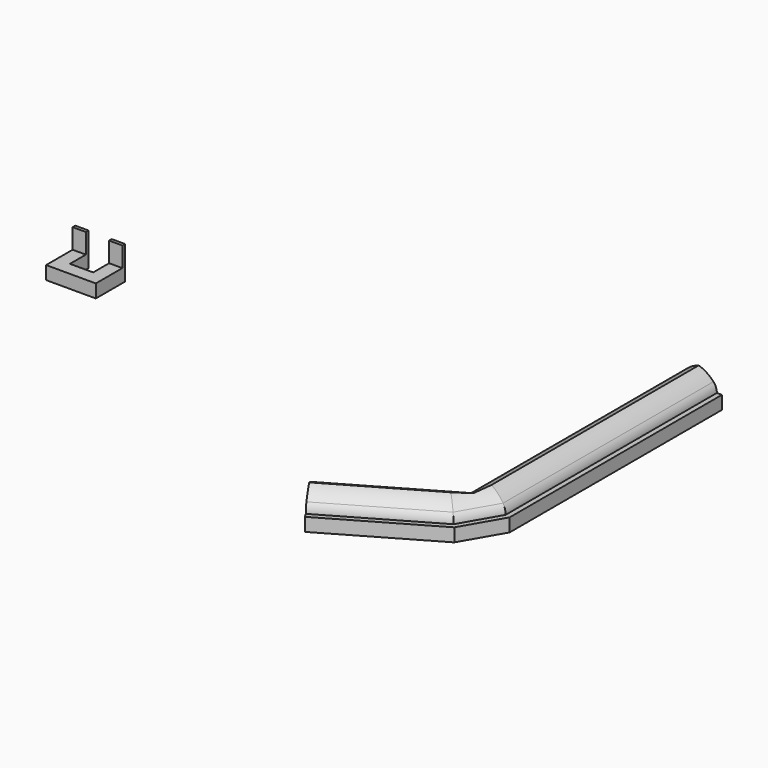
from build123d import *

# Parameters (mm, degrees)
F0_W         = 7
F0_H         = 40
F1_DEPTH     = 5
F2_T1_DEPTH  = 32
F2_T3_DEPTH  = 42.8011414996
F2_T5_DEPTH  = 65
F2_T10_DEPTH = 65
F2_T15_DEPTH = 42.8011414996
F2_T21_DEPTH = 65
F2_T25_DEPTH = 42.8011414996
F3_R         = 2
F4_DEPTH     = 2
F0_W_2       = 2
F0_H_2       = 0.5
F5_DEPTH     = 5


# Not quite as in the source:
# - a fillet or chamfer that OpenCascade refuses, or shapes differently, is made with other operations: its cross-section is extruded or revolved along the edge and cut away or added


with BuildPart() as f1:
    # F0 (on Top) → F1 (new body)
    with BuildSketch(Plane.XY):
        Polygon((30.4447099417, -16.7805150867), (26.9447099417, -10.7183372602), (11.5284691868, -19.61890801), (15.0284691868, -25.6810858365), align=None)
        Polygon((33.9447099417, -10.7183372602), (26.9447099417, -10.7183372602), (30.4447099417, -16.7805150867), align=None)
        with Locations((30.4447099417, 9.2816627398)):
            Rectangle(F0_W, F0_H)
    extrude(amount=F1_DEPTH)

    # F2: fillet of radius 5 on 5 edges, made by hand

    # F2_s2 → F2_t1 (cut)
    with BuildSketch(Plane(origin=(-5.9049986914, -10.2277577521, 0), x_dir=(0, 0, 1), z_dir=(0.5, 0.8660254038, 0))):
        with BuildLine():
            ThreePointArc((0, 34.7561497637), (3.5355339059, 33.2916836697), (5, 29.7561497637))
            Line((5, 29.7561497637), (5, 34.7561497637))
            Line((5, 34.7561497637), (0, 34.7561497637))
        make_face()
    extrude(amount=F2_T1_DEPTH, mode=Mode.SUBTRACT)

    # F2_s4 → F2_t3 (cut)
    with BuildSketch(Plane(origin=(-10.6742020228, -6.1627534112, 0), x_dir=(0, 0, 1), z_dir=(0.8660254038, 0.5, 0))):
        with BuildLine():
            ThreePointArc((0, 29.7547073245), (3.5355339059, 28.2902412305), (5, 24.7547073245))
            Line((5, 24.7547073245), (5, 29.7547073245))
            Line((5, 29.7547073245), (0, 29.7547073245))
        make_face()
    extrude(amount=F2_T3_DEPTH, mode=Mode.SUBTRACT)

    # F2_s6 → F2_t5 (cut)
    with BuildSketch(Plane.XZ.offset(-41.7816627398)):
        with BuildLine():
            ThreePointArc((33.9447099417, 0), (32.4802438477, 3.5355339059), (28.9447099417, 5))
            Line((28.9447099417, 5), (33.9447099417, 5))
            Line((33.9447099417, 5), (33.9447099417, 0))
        make_face()
    extrude(amount=F2_T5_DEPTH, mode=Mode.SUBTRACT)


with BuildPart() as f2_tool8:
    # F2_s9 → F2_t10 (new body)
    with BuildSketch(Plane.XZ.offset(-41.7816627398)):
        with BuildLine():
            ThreePointArc((26.9447099417, 0), (28.4091760358, 3.5355339059), (31.9447099417, 5))
            Line((31.9447099417, 5), (26.9447099417, 5))
            Line((26.9447099417, 5), (26.9447099417, 0))
        make_face()
    extrude(amount=F2_T10_DEPTH)

    split(bisect_by=Plane(origin=(11.3773536623, -19.7061545987, 0), x_dir=(0, 0, 1), z_dir=(-0.5, 0.8660254038, 0)), keep=Keep.TOP)


with BuildPart() as f1_1:
    add(f1.part)

    # F2_t7: cut F2_tool8
    add(f2_tool8.part, mode=Mode.SUBTRACT)


with BuildPart() as f2_tool13:
    # F2_s14 → F2_t15 (new body)
    with BuildSketch(Plane(origin=(26.3926738268, 15.2378173385, 0), x_dir=(0, 0, 1), z_dir=(-0.8660254038, -0.5, 0))):
        with BuildLine():
            ThreePointArc((0, -22.7547073245), (3.5355339059, -24.2191734186), (5, -27.7547073245))
            Line((5, -27.7547073245), (5, -22.7547073245))
            Line((5, -22.7547073245), (0, -22.7547073245))
        make_face()
    extrude(amount=F2_T15_DEPTH)

    split(bisect_by=Plane.YZ.offset(26.9447099417), keep=Keep.BOTTOM)


with BuildPart() as f1_2:
    add(f1_1.part)

    # F2_t12: cut F2_tool13
    add(f2_tool13.part, mode=Mode.SUBTRACT)


with BuildPart() as f2_tool19:
    # F2_s20 → F2_t21 (new body)
    with BuildSketch(Plane.XZ.offset(-41.7816627398)):
        with BuildLine():
            ThreePointArc((26.9447099417, 0), (28.4091760358, 3.5355339059), (31.9447099417, 5))
            Line((31.9447099417, 5), (26.9447099417, 5))
            Line((26.9447099417, 5), (26.9447099417, 0))
        make_face()
    extrude(amount=F2_T21_DEPTH)

    split(bisect_by=Plane(origin=(11.3773536623, -19.7061545987, 0), x_dir=(0, 0, 1), z_dir=(0.5, -0.8660254038, 0)), keep=Keep.TOP)


with BuildPart() as f2_tool23:
    # F2_s24 → F2_t25 (new body)
    with BuildSketch(Plane(origin=(26.3926738268, 15.2378173385, 0), x_dir=(0, 0, 1), z_dir=(-0.8660254038, -0.5, 0))):
        with BuildLine():
            ThreePointArc((0, -22.7547073245), (3.5355339059, -24.2191734186), (5, -27.7547073245))
            Line((5, -27.7547073245), (5, -22.7547073245))
            Line((5, -22.7547073245), (0, -22.7547073245))
        make_face()
    extrude(amount=F2_T25_DEPTH)

    split(bisect_by=Plane.YZ.offset(26.9447099417), keep=Keep.TOP)


with BuildPart() as f2_tool19_1:
    add(f2_tool19.part)

    # F2_t27: intersect F2_tool23
    add(f2_tool23.part, mode=Mode.INTERSECT)


with BuildPart() as f1_3:
    add(f1_2.part)

    # F2_t17: cut F2_tool19
    add(f2_tool19_1.part, mode=Mode.SUBTRACT)

    # F3
    f3_edges = [f1_3.edges().sort_by_distance(p)[0] for p in [
        (13.278469, -22.649997, 0),
        (22.73659, -21.2308, 0),
        (19.23659, -15.168623, 0),
        (26.94471, 9.281663, 0),
        (33.94471, 9.281663, 0),
        (32.19471, -13.749426, 0),
        (30.44471, 29.281663, 0),
    ]]
    fillet(f3_edges, radius=F3_R)

    # F0 (on Top) → F4 (join)
    with BuildSketch(Plane.XY):
        with Locations((30.4447099417, 9.2816627398)):
            Rectangle(F0_W, F0_H)
        Polygon((30.4447099417, -16.7805150867), (26.9447099417, -10.7183372602), (11.5284691868, -19.61890801), (15.0284691868, -25.6810858365), align=None)
        Polygon((33.9447099417, -10.7183372602), (26.9447099417, -10.7183372602), (30.4447099417, -16.7805150867), align=None)
    extrude(amount=F4_DEPTH)


with BuildPart() as f4:
    # F0 (on Top) → F4, piece 2 (new body)
    with BuildSketch(Plane.XY):
        Polygon((-46.8554012775, 10.416974891), (-48.8554012775, 10.416974891), (-48.8554012775, 5.416974891), (-41.3554012775, 5.416974891), (-41.3554012775, 10.416974891), (-43.3554012775, 10.416974891), (-43.3554012775, 7.416974891), (-46.8554012775, 7.416974891), align=None)
    extrude(amount=F4_DEPTH)

    # F0 (on Top) → F5 (join)
    with BuildSketch(Plane.XY):
        with Locations((-47.8554012775, 10.666974891)):
            Rectangle(F0_W_2, F0_H_2)
        with Locations((-42.3554012775, 10.666974891)):
            Rectangle(F0_W_2, F0_H_2)
    extrude(amount=F5_DEPTH)


solid = Compound([f1_3.part, f4.part])
